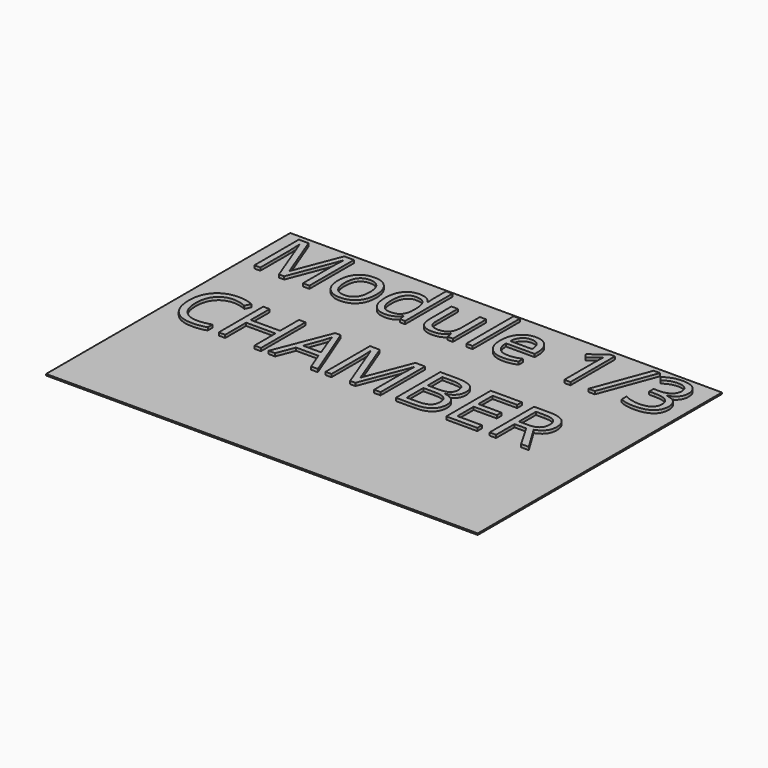
from build123d import *

# Parameters (mm, degrees)
F0_W         = 297
F0_H         = 210
F1_DEPTH     = 1
F2_TEXT_SIZE = 53.5855380197
F3_DEPTH     = 2


# Not quite as in the source:
# - Text() gives the source's letters only with a copy of the font that has no kerning and outlines rounded to 1/6400 em; it was checked with that copy


with BuildPart() as f1:
    # F0 (on Top) → F1 (new body)
    with BuildSketch(Plane.XY):
        with Locations((-47.4010080695, 34.3840229511)):
            Rectangle(F0_W, F0_H)
    extrude(amount=F1_DEPTH)

    # F2 (on face) → F3 (join)
    with BuildSketch(Plane.XY.offset(1)):
        with Locations((-190.3507038951, 94.9954763055)):
            Text('Module 1/3', F2_TEXT_SIZE, font='Open Sans', text_align=(TextAlign.LEFT, TextAlign.BOTTOM))
        with Locations((-190.3507038951, 22.1191445986)):
            Text('CHAMBER', F2_TEXT_SIZE, font='Open Sans', text_align=(TextAlign.LEFT, TextAlign.BOTTOM))
    extrude(amount=F3_DEPTH)


solid = f1.part
